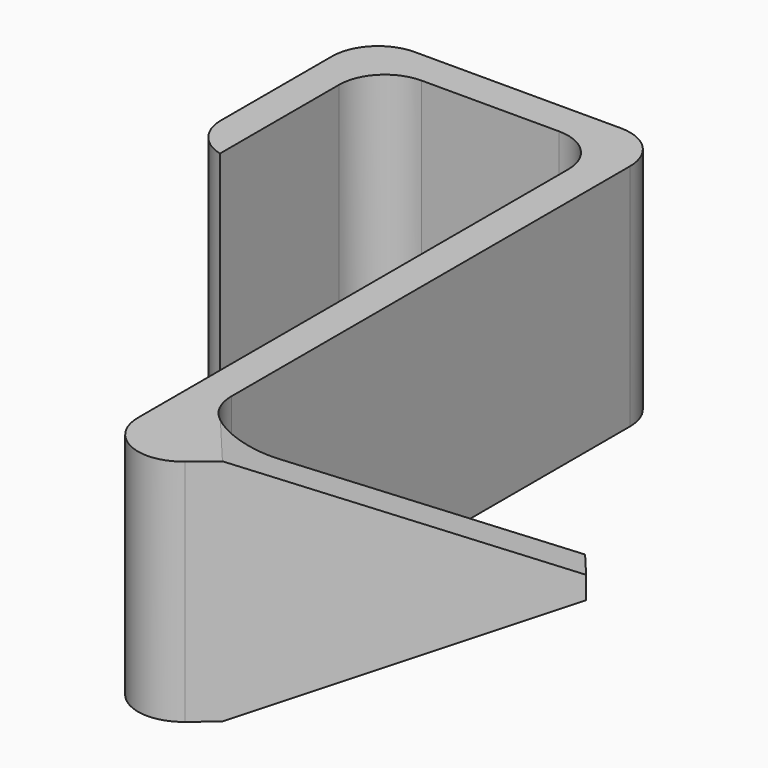
from build123d import *

# Parameters (mm, degrees)
F1_DEPTH     = 25.4
F2_T1_DEPTH  = 25.4
F2_T3_DEPTH  = 25.4
F2_T5_DEPTH  = 25.4
F2_T7_DEPTH  = 50.8
F2_T9_DEPTH  = 50.8
F2_T11_DEPTH = 49.9934442484
F3_SIZE2     = 11.4636064984
F3_SIZE      = 31.496
F3_2_SIZE2   = 11.4636064984
F3_2_SIZE    = 31.496
F4_T1_DEPTH  = 50.8
F5_T1_DEPTH  = 68.1227876391


# Not quite as in the source:
# - a fillet or chamfer that OpenCascade refuses, or shapes differently, is made with other operations: its cross-section is extruded or revolved along the edge and cut away or added


with BuildPart() as f1:
    # F0 (on Top) → F1 (new body)
    with BuildSketch(Plane.XY):
        Polygon((33.02, 0), (0, 0), (0, -25.4), (3.81, -25.4), (3.81, -3.81), (29.21, -3.81), (29.21, -76.2), (33.02, -76.2), (33.02, -71.2263982276), align=None)
        Polygon((61.7030253754, -47.1584822141), (33.02, -71.2263982276), (33.02, -76.2), (64.1520461684, -50.0771115423), align=None)
    extrude(amount=F1_DEPTH)

    # F2: fillet of radius 5.08 on 6 edges, made by hand

    # F2_s2 → F2_t1 (join)
    with BuildSketch(Plane.XY):
        with BuildLine():
            ThreePointArc((3.81, -8.89), (5.2978975516, -5.2978975516), (8.89, -3.81))
            Line((8.89, -3.81), (3.81, -3.81))
            Line((3.81, -3.81), (3.81, -8.89))
        make_face()
    extrude(amount=F2_T1_DEPTH)

    # F2_s4 → F2_t3 (join)
    with BuildSketch(Plane.XY):
        with BuildLine():
            ThreePointArc((24.13, -3.81), (27.7221024484, -5.2978975516), (29.21, -8.89))
            Line((29.21, -8.89), (29.21, -3.81))
            Line((29.21, -3.81), (24.13, -3.81))
        make_face()
    extrude(amount=F2_T3_DEPTH)

    # F2_s6 → F2_t5 (join)
    with BuildSketch(Plane.XY):
        with BuildLine():
            ThreePointArc((33.02, -60.3323030715), (35.9530992304, -64.9363466296), (41.3653610572, -64.2238088425))
            Line((41.3653610572, -64.2238088425), (33.02, -71.2263982276))
            Line((33.02, -71.2263982276), (33.02, -60.3323030715))
        make_face()
    extrude(amount=F2_T5_DEPTH)

    # F2_s8 → F2_t7 (cut)
    with BuildSketch(Plane.XY.offset(-12.7)):
        with BuildLine():
            ThreePointArc((27.94, 0), (31.5321024484, -1.4878975516), (33.02, -5.08))
            Line((33.02, -5.08), (33.02, 0))
            Line((33.02, 0), (27.94, 0))
        make_face()
    extrude(amount=F2_T7_DEPTH, mode=Mode.SUBTRACT)

    # F2_s10 → F2_t9 (cut)
    with BuildSketch(Plane.XY.offset(-12.7)):
        with BuildLine():
            ThreePointArc((5.08, 0), (1.4878975516, -1.4878975516), (0, -5.08))
            Line((0, -5.08), (0, 0))
            Line((0, 0), (5.08, 0))
        make_face()
    extrude(amount=F2_T9_DEPTH, mode=Mode.SUBTRACT)

    # F2_s12 → F2_t11 (cut)
    with BuildSketch(Plane.XY.offset(-12.2967221242)):
        with BuildLine():
            ThreePointArc((3.81, -25.4), (1.0639073716, -23.5921631237), (0, -20.4813111503))
            Line((0, -20.4813111503), (0, -25.4))
            Line((0, -25.4), (3.81, -25.4))
        make_face()
    extrude(amount=F2_T11_DEPTH, mode=Mode.SUBTRACT)

    # F3
    f3_edges = [f1.edges().sort_by_distance(p)[0] for p in [
        (62.927536, -48.617797, 25.4),
    ]]
    f3_side = f1.faces().sort_by_distance((30.827761, -2.192239, 25.4))[0]
    chamfer(f3_edges, length=F3_SIZE, length2=F3_SIZE2, reference=f3_side)

    # F3#2
    f3_2_edges = [f1.edges().sort_by_distance(p)[0] for p in [
        (62.927536, -48.617797, 0),
    ]]
    f3_2_side = f1.faces().sort_by_distance((30.827761, -2.192239, 0))[0]
    chamfer(f3_2_edges, length=F3_2_SIZE, length2=F3_2_SIZE2, reference=f3_2_side)

    # F4: fillet of radius 5.08 on 1 edges, made by hand

    # F4_s2 → F4_t1 (cut)
    with BuildSketch(Plane.XY.offset(-12.7)):
        with BuildLine():
            ThreePointArc((34.29, -76.2), (30.6978975516, -74.7121024484), (29.21, -71.12))
            Line((29.21, -71.12), (29.21, -76.2))
            Line((29.21, -76.2), (34.29, -76.2))
        make_face()
    extrude(amount=F4_T1_DEPTH, mode=Mode.SUBTRACT)

    # F5: fillet of radius 5.08 on 1 edges, made by hand

    # F5_s2 → F5_t1 (cut)
    with BuildSketch(Plane.XY.offset(-21.3613938196)):
        with BuildLine():
            ThreePointArc((37.5553610572, -72.3943802096), (32.1430992304, -73.1069179967), (29.21, -68.5028744386))
            Line((29.21, -68.5028744386), (28.702, -68.5028744386))
            ThreePointArc((28.702, -68.5028744386), (28.702, -71.12), (33.0571094194, -76.5702958467))
            Line((33.0571094194, -76.5702958467), (33.495726487, -76.4639649832))
            Line((33.495726487, -76.4639649832), (37.8818971629, -72.7835307867))
            Line((37.8818971629, -72.7835307867), (37.5553610572, -72.3943802096))
        make_face()
    extrude(amount=F5_T1_DEPTH, mode=Mode.SUBTRACT)


solid = f1.part
